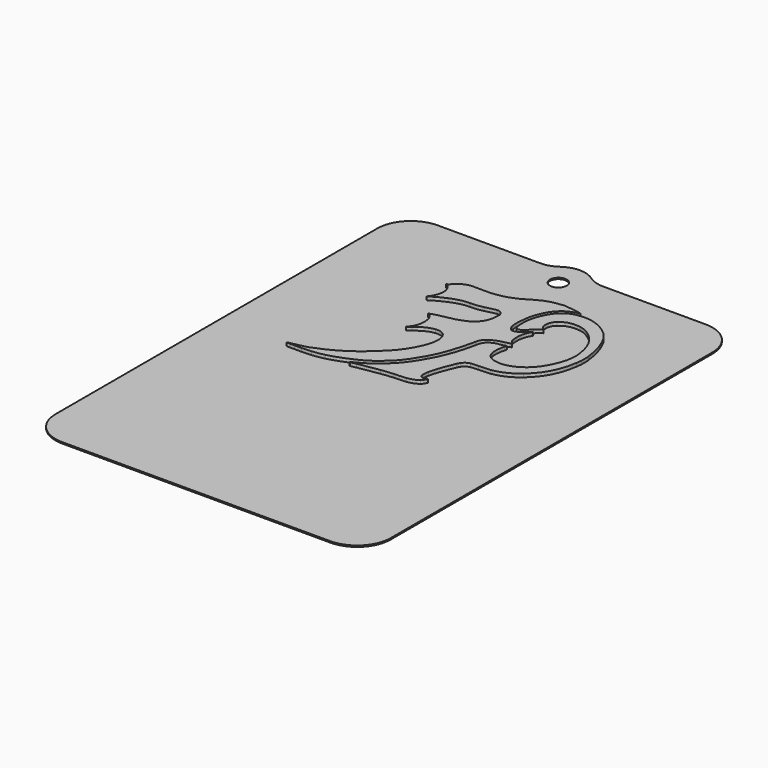
from build123d import *

# Parameters (mm, degrees)
F0_R     = 2.5
F1_DEPTH = 0.2
F3_DEPTH = 1


# Not quite as in the source:
# - ends of sketch curves that miss each other by under 0.0002 mm in the source are joined


with BuildPart() as f1:
    # F0 (on Top) → F1 (new body, symmetric)
    with BuildSketch(Plane.XY):
        with BuildLine():
            Line((-9.3273790531, 70), (-40, 70))
            ThreePointArc((-40, 70), (-47.0710678119, 67.0710678119), (-50, 60))
            Line((-50, 60), (-50, -60))
            ThreePointArc((-50, -60), (-47.0710678119, -67.0710678119), (-40, -70))
            Line((-40, -70), (40, -70))
            ThreePointArc((40, -70), (47.0710678119, -67.0710678119), (50, -60))
            Line((50, -60), (50, 60))
            ThreePointArc((50, 60), (47.0710678119, 67.0710678119), (40, 70))
            Line((40, 70), (9.3273790531, 70))
            ThreePointArc((9.3273790531, 70), (6.8778893103, 70.3842268941), (4.6636895265, 71.5))
            ThreePointArc((4.6636895265, 71.5), (0, 73), (-4.6636895265, 71.5))
            ThreePointArc((-4.6636895265, 71.5), (-6.8778893103, 70.3842268941), (-9.3273790531, 70))
        make_face()
        with Locations((0, 65)):
            Circle(F0_R, mode=Mode.SUBTRACT)
    extrude(amount=F1_DEPTH, both=True)

    # F2 (on face) → F3 (join)
    with BuildSketch(Plane.XY.offset(0.2)):
        with BuildLine():
            add(Edge.make_bspline(
                [(10.0940918419, 55.33162), (10.3944688419, 55.204597), (10.7172378419, 55.217338), (11.0315138419, 55.192628)],
                knots=[0, 0, 0, 0, 1, 1, 1, 1], degree=3))
            add(Edge.make_bspline(
                [(9.9539408419, 55.33162), (10.0006588419, 55.33162), (10.0473758419, 55.33162), (10.0940918419, 55.33162)],
                knots=[0, 0, 0, 0, 1, 1, 1, 1], degree=3))
            add(Edge.make_bspline(
                [(9.2528058419, 55.33162), (9.4867748419, 55.33162), (9.7203578419, 55.33162), (9.9539408419, 55.33162)],
                knots=[0, 0, 0, 0, 1, 1, 1, 1], degree=3))
            add(Edge.make_bspline(
                [(9.1829238419, 55.33162), (9.2060898419, 55.33162), (9.2296408419, 55.33162), (9.2528058419, 55.33162)],
                knots=[0, 0, 0, 0, 1, 1, 1, 1], degree=3))
            add(Edge.make_bspline(
                [(8.5254158419, 55.196103), (8.7489618419, 55.211932), (8.9786838419, 55.213091), (9.1829238419, 55.33162)],
                knots=[0, 0, 0, 0, 1, 1, 1, 1], degree=3))
            add(Edge.make_bspline(
                [(4.2919618419, 54.221617), (5.6490608419, 54.787622), (7.0652308419, 55.090315), (8.5254158419, 55.196103)],
                knots=[0, 0, 0, 0, 1, 1, 1, 1], degree=3))
            add(Edge.make_bspline(
                [(0.2326328419, 52.031726), (1.5545978419, 52.820503), (2.8676828419, 53.627427), (4.2919618419, 54.221617)],
                knots=[0, 0, 0, 0, 1, 1, 1, 1], degree=3))
            add(Edge.make_bspline(
                [(-9.8682011581, 49.538756), (-6.2826021581, 49.433354), (-2.8873441581, 50.170396), (0.2326328419, 52.031726)],
                knots=[0, 0, 0, 0, 1, 1, 1, 1], degree=3))
            add(Edge.make_bspline(
                [(-12.9140491581, 49.590491), (-11.8997961581, 49.615587), (-10.8839981581, 49.568484), (-9.8682011581, 49.538756)],
                knots=[0, 0, 0, 0, 1, 1, 1, 1], degree=3))
            add(Edge.make_bspline(
                [(-16.5571751581, 48.373542), (-15.5023831581, 49.256525), (-14.2402611581, 49.557674), (-12.9140491581, 49.590491)],
                knots=[0, 0, 0, 0, 1, 1, 1, 1], degree=3))
            add(Edge.make_bspline(
                [(-18.6961021581, 46.557384), (-17.8644691581, 47.043469), (-17.2695081581, 47.777808), (-16.5571751581, 48.373542)],
                knots=[0, 0, 0, 0, 1, 1, 1, 1], degree=3))
            add(Edge.make_bspline(
                [(-17.4463361581, 45.553555), (-17.7463261581, 46.02188), (-18.2092461581, 46.269363), (-18.6961021581, 46.557384)],
                knots=[0, 0, 0, 0, 1, 1, 1, 1], degree=3))
            add(Edge.make_bspline(
                [(-17.0818691581, 41.268751), (-16.6058231581, 42.730481), (-16.5726191581, 44.188734), (-17.4463361581, 45.553555)],
                knots=[0, 0, 0, 0, 1, 1, 1, 1], degree=3))
            add(Edge.make_bspline(
                [(-18.4300881581, 38.924039), (-17.8135051581, 39.617067), (-17.3610101581, 40.410864), (-17.0818691581, 41.268751)],
                knots=[0, 0, 0, 0, 1, 1, 1, 1], degree=3))
            add(Edge.make_bspline(
                [(-18.1783581581, 39.002415), (-18.2420631581, 38.957243), (-18.2972741581, 38.882728), (-18.4300881581, 38.924039)],
                knots=[0, 0, 0, 0, 1, 1, 1, 1], degree=3))
            add(Edge.make_bspline(
                [(-13.9483791581, 41.308132), (-15.4317291581, 40.67572), (-16.8583241581, 39.940608), (-18.1783581581, 39.002415)],
                knots=[0, 0, 0, 0, 1, 1, 1, 1], degree=3))
            add(Edge.make_bspline(
                [(-8.3779011581, 42.584153), (-10.3419311581, 42.619673), (-12.1650391581, 42.06834), (-13.9483791581, 41.308132)],
                knots=[0, 0, 0, 0, 1, 1, 1, 1], degree=3))
            add(Edge.make_bspline(
                [(-4.5328511581, 43.025065), (-5.8026941581, 42.745151), (-7.0806461581, 42.560987), (-8.3779011581, 42.584153)],
                knots=[0, 0, 0, 0, 1, 1, 1, 1], degree=3))
            add(Edge.make_bspline(
                [(-1.3754241581, 43.768671), (-2.4445011581, 43.591071), (-3.4765151581, 43.257876), (-4.5328511581, 43.025065)],
                knots=[0, 0, 0, 0, 1, 1, 1, 1], degree=3))
            add(Edge.make_bspline(
                [(0.7086788419, 42.071814), (0.6426578419, 43.163671), (-0.3221761581, 43.943955), (-1.3754241581, 43.768671)],
                knots=[0, 0, 0, 0, 1, 1, 1, 1], degree=3))
            add(Edge.make_bspline(
                [(0.5662128419, 40.378047), (0.6117708419, 40.942507), (0.7434268419, 41.498088), (0.7086788419, 42.071814)],
                knots=[0, 0, 0, 0, 1, 1, 1, 1], degree=3))
            add(Edge.make_bspline(
                [(-0.8874091581, 36.858468), (0.0237588419, 37.853803), (0.4588798419, 39.044499), (0.5662128419, 40.378047)],
                knots=[0, 0, 0, 0, 1, 1, 1, 1], degree=3))
            add(Edge.make_bspline(
                [(-3.3726571581, 35.005246), (-2.4024181581, 35.434962), (-1.6009001581, 36.078956), (-0.8874091581, 36.858468)],
                knots=[0, 0, 0, 0, 1, 1, 1, 1], degree=3))
            add(Edge.make_bspline(
                [(-5.8926531581, 34.088287), (-5.0316771581, 34.334997), (-4.1938661581, 34.641551), (-3.3726571581, 35.005246)],
                knots=[0, 0, 0, 0, 1, 1, 1, 1], degree=3))
            add(Edge.make_bspline(
                [(-10.8380541581, 33.021912), (-9.1917751581, 33.387537), (-7.5180831581, 33.622665), (-5.8926531581, 34.088287)],
                knots=[0, 0, 0, 0, 1, 1, 1, 1], degree=3))
            add(Edge.make_bspline(
                [(-12.7812341581, 32.350505), (-12.1495951581, 32.687946), (-11.4986501581, 32.875585), (-10.8380541581, 33.021912)],
                knots=[0, 0, 0, 0, 1, 1, 1, 1], degree=3))
            add(Edge.make_bspline(
                [(-11.0044581581, 30.218913), (-11.2191231581, 31.210001), (-11.8082931581, 31.929669), (-12.7812341581, 32.350505)],
                knots=[0, 0, 0, 0, 1, 1, 1, 1], degree=3))
            add(Edge.make_bspline(
                [(-12.5457211581, 24.119495), (-10.9013721581, 25.859207), (-10.5087211581, 27.931728), (-11.0044581581, 30.218913)],
                knots=[0, 0, 0, 0, 1, 1, 1, 1], degree=3))
            add(Edge.make_bspline(
                [(-12.5769951581, 23.968921), (-12.6275721581, 24.070462), (-12.5727451581, 24.091311), (-12.5457211581, 24.119495)],
                knots=[0, 0, 0, 0, 1, 1, 1, 1], degree=3))
            add(Edge.make_bspline(
                [(-11.5044411581, 24.802099), (-11.8654341581, 24.534153), (-12.2152301581, 24.250379), (-12.5769951581, 23.968921)],
                knots=[0, 0, 0, 0, 1, 1, 1, 1], degree=3))
            add(Edge.make_bspline(
                [(-6.4984251581, 27.232909), (-8.4358151581, 26.997009), (-9.9859581581, 25.92909), (-11.5044411581, 24.802099)],
                knots=[0, 0, 0, 0, 1, 1, 1, 1], degree=3))
            add(Edge.make_bspline(
                [(-2.7190101581, 24.706735), (-3.2228551581, 26.661885), (-4.5575611581, 27.469195), (-6.4984251581, 27.232909)],
                knots=[0, 0, 0, 0, 1, 1, 1, 1], degree=3))
            add(Edge.make_bspline(
                [(-2.7722901581, 21.715325), (-2.5653471581, 22.709502), (-2.4703691581, 23.741901), (-2.7190101581, 24.706735)],
                knots=[0, 0, 0, 0, 1, 1, 1, 1], degree=3))
            add(Edge.make_bspline(
                [(-5.7428511581, 15.177312), (-4.4170251581, 17.193077), (-3.2742041581, 19.308453), (-2.7722901581, 21.715325)],
                knots=[0, 0, 0, 0, 1, 1, 1, 1], degree=3))
            add(Edge.make_bspline(
                [(-11.4341741581, 9.089477), (-9.3361711581, 10.922622), (-7.2918361581, 12.822175), (-5.7428511581, 15.177312)],
                knots=[0, 0, 0, 0, 1, 1, 1, 1], degree=3))
            add(Edge.make_bspline(
                [(-14.5618731581, 6.584538), (-13.4534141581, 7.317333), (-12.4407051581, 8.209968), (-11.4341741581, 9.089477)],
                knots=[0, 0, 0, 0, 1, 1, 1, 1], degree=3))
            add(Edge.make_bspline(
                [(-18.2134931581, 4.309321), (-16.9239591581, 4.957948), (-15.7556561581, 5.79576), (-14.5618731581, 6.584538)],
                knots=[0, 0, 0, 0, 1, 1, 1, 1], degree=3))
            add(Edge.make_bspline(
                [(-21.1991111581, 2.868823), (-20.1566731581, 3.238313), (-19.2018781581, 3.812426), (-18.2134931581, 4.309321)],
                knots=[0, 0, 0, 0, 1, 1, 1, 1], degree=3))
            add(Edge.make_bspline(
                [(-24.0897521581, 1.666931), (-23.0890121581, 1.970396), (-22.1859521581, 2.519027), (-21.1991111581, 2.868823)],
                knots=[0, 0, 0, 0, 1, 1, 1, 1], degree=3))
            add(Edge.make_bspline(
                [(-25.6128691581, 1.290496), (-25.1070931581, 1.424467), (-24.5897361581, 1.515585), (-24.0897521581, 1.666931)],
                knots=[0, 0, 0, 0, 1, 1, 1, 1], degree=3))
            add(Edge.make_bspline(
                [(-29.4328231581, 0.475463), (-28.1529421581, 0.71561), (-26.8734461581, 0.956916), (-25.6128691581, 1.290496)],
                knots=[0, 0, 0, 0, 1, 1, 1, 1], degree=3))
            add(Edge.make_bspline(
                [(-29.4328231581, 0.475463), (-29.0664261581, 0.330298), (-28.6830401581, 0.464657), (-28.3116241581, 0.404814)],
                knots=[0, 0, 0, 0, 1, 1, 1, 1], degree=3))
            Line((-28.3116241581, 0.404814), (-27.0529771581, 0.404042))
            add(Edge.make_bspline(
                [(-26.6325271581, 0.404042), (-26.7726771581, 0.404042), (-26.9128271581, 0.404042), (-27.0529771581, 0.404042)],
                knots=[0, 0, 0, 0, 1, 1, 1, 1], degree=3))
            add(Edge.make_bspline(
                [(-25.9313911581, 0.404042), (-26.1653601581, 0.404042), (-26.3989431581, 0.404042), (-26.6325271581, 0.404042)],
                knots=[0, 0, 0, 0, 1, 1, 1, 1], degree=3))
            add(Edge.make_bspline(
                [(-24.9503421581, 0.404042), (-25.2773581581, 0.404042), (-25.6043751581, 0.404042), (-25.9313911581, 0.404042)],
                knots=[0, 0, 0, 0, 1, 1, 1, 1], degree=3))
            add(Edge.make_bspline(
                [(-22.0855691581, 0.557318), (-23.0384341581, 0.460024), (-23.9928441581, 0.402883), (-24.9503421581, 0.404042)],
                knots=[0, 0, 0, 0, 1, 1, 1, 1], degree=3))
            add(Edge.make_bspline(
                [(-18.5343311581, 1.110968), (-19.6949121581, 0.813681), (-20.8917851581, 0.679708), (-22.0855691581, 0.557318)],
                knots=[0, 0, 0, 0, 1, 1, 1, 1], degree=3))
            add(Edge.make_bspline(
                [(-10.4612321581, 4.162221), (-13.0646231581, 2.913227), (-15.7359661581, 1.827161), (-18.5343311581, 1.110968)],
                knots=[0, 0, 0, 0, 1, 1, 1, 1], degree=3))
            add(Edge.make_bspline(
                [(-4.8602541581, 8.231975), (-6.5744851581, 6.655192), (-8.3562801581, 5.171842), (-10.4612321581, 4.162221)],
                knots=[0, 0, 0, 0, 1, 1, 1, 1], degree=3))
            add(Edge.make_bspline(
                [(0.3469148419, 15.298543), (-1.1252391581, 12.748818), (-2.6699771581, 10.246968), (-4.8602541581, 8.231975)],
                knots=[0, 0, 0, 0, 1, 1, 1, 1], degree=3))
            add(Edge.make_bspline(
                [(2.8645938419, 21.104535), (2.1846938419, 19.099193), (1.4044088419, 17.129758), (0.3469148419, 15.298543)],
                knots=[0, 0, 0, 0, 1, 1, 1, 1], degree=3))
            add(Edge.make_bspline(
                [(4.7807488419, 28.180755), (4.2896448419, 25.779674), (3.6502828419, 23.421835), (2.8645938419, 21.104535)],
                knots=[0, 0, 0, 0, 1, 1, 1, 1], degree=3))
            add(Edge.make_bspline(
                [(6.2444078419, 30.588786), (5.4015788419, 30.001159), (4.9772678419, 29.142499), (4.7807488419, 28.180755)],
                knots=[0, 0, 0, 0, 1, 1, 1, 1], degree=3))
            add(Edge.make_bspline(
                [(9.5157318419, 32.030438), (8.3466578419, 31.73508), (7.2443758419, 31.285674), (6.2444078419, 30.588786)],
                knots=[0, 0, 0, 0, 1, 1, 1, 1], degree=3))
            add(Edge.make_bspline(
                [(11.5388328419, 32.54934), (10.8913638419, 32.270585), (10.1906138419, 32.201089), (9.5157318419, 32.030438)],
                knots=[0, 0, 0, 0, 1, 1, 1, 1], degree=3))
            add(Edge.make_bspline(
                [(11.6554318419, 33.103376), (12.0129498419, 32.764777), (12.0005948419, 32.74779), (11.5388328419, 32.54934)],
                knots=[0, 0, 0, 0, 1, 1, 1, 1], degree=3))
            add(Edge.make_bspline(
                [(11.0071888419, 34.327661), (11.0901988419, 33.855476), (11.2983008419, 33.442362), (11.6554318419, 33.103376)],
                knots=[0, 0, 0, 0, 1, 1, 1, 1], degree=3))
            add(Edge.make_bspline(
                [(11.9492438419, 40.017054), (10.8600898419, 38.25186), (10.6531468419, 36.335705), (11.0071888419, 34.327661)],
                knots=[0, 0, 0, 0, 1, 1, 1, 1], degree=3))
            add(Edge.make_bspline(
                [(12.1040658419, 40.391945), (12.1110138419, 40.195427), (12.0079298419, 40.112032), (11.9492438419, 40.017054)],
                knots=[0, 0, 0, 0, 1, 1, 1, 1], degree=3))
            add(Edge.make_bspline(
                [(11.4863248419, 39.735982), (11.6909508419, 39.926323), (11.8716408419, 40.143305), (12.1040658419, 40.391945)],
                knots=[0, 0, 0, 0, 1, 1, 1, 1], degree=3))
            add(Edge.make_bspline(
                [(8.9420048419, 38.025998), (9.9168768419, 38.407454), (10.7284338419, 39.02944), (11.4863248419, 39.735982)],
                knots=[0, 0, 0, 0, 1, 1, 1, 1], degree=3))
            add(Edge.make_bspline(
                [(6.7922668419, 38.884658), (7.2076978419, 38.142597), (7.8208058419, 37.587016), (8.9420048419, 38.025998)],
                knots=[0, 0, 0, 0, 1, 1, 1, 1], degree=3))
            add(Edge.make_bspline(
                [(6.5173728419, 39.716678), (6.5733558419, 39.425953), (6.6467128419, 39.145267), (6.7922668419, 38.884658)],
                knots=[0, 0, 0, 0, 1, 1, 1, 1], degree=3))
            add(Edge.make_bspline(
                [(6.6289518419, 44.590652), (6.4297298419, 42.977962), (6.2030978419, 41.349443), (6.5173728419, 39.716678)],
                knots=[0, 0, 0, 0, 1, 1, 1, 1], degree=3))
            add(Edge.make_bspline(
                [(8.1408718419, 49.376985), (7.3683108419, 47.868925), (6.8358948419, 46.267818), (6.6289518419, 44.590652)],
                knots=[0, 0, 0, 0, 1, 1, 1, 1], degree=3))
            add(Edge.make_bspline(
                [(13.1163888419, 53.981856), (10.7983158419, 53.173002), (9.2427678419, 51.528267), (8.1408718419, 49.376985)],
                knots=[0, 0, 0, 0, 1, 1, 1, 1], degree=3))
            add(Edge.make_bspline(
                [(15.1031968419, 54.423927), (14.4020608419, 54.402692), (13.7592248419, 54.205787), (13.1163888419, 53.981856)],
                knots=[0, 0, 0, 0, 1, 1, 1, 1], degree=3))
            add(Edge.make_bspline(
                [(14.7896938419, 54.609635), (14.8916218419, 54.583381), (15.0255928419, 54.58647), (15.1031968419, 54.423927)],
                knots=[0, 0, 0, 0, 1, 1, 1, 1], degree=3))
            add(Edge.make_bspline(
                [(11.0315138419, 55.192628), (12.2990408419, 55.092631), (13.5553698419, 54.924683), (14.7896938419, 54.609635)],
                knots=[0, 0, 0, 0, 1, 1, 1, 1], degree=3))
        make_face()
        with BuildLine():
            add(Edge.make_bspline(
                [(30.0000158419, 35.937262), (29.8228008419, 35.509091), (29.8656578419, 35.046557), (29.8042688419, 34.601398)],
                knots=[0, 0, 0, 0, 1, 1, 1, 1], degree=3))
            add(Edge.make_bspline(
                [(30.0000158419, 36.363504), (30.0000158419, 36.221423), (30.0000158419, 36.079343), (30.0000158419, 35.937262)],
                knots=[0, 0, 0, 0, 1, 1, 1, 1], degree=3))
            add(Edge.make_bspline(
                [(30.0000158419, 36.505584), (30.0000158419, 36.458095), (30.0000158419, 36.410993), (30.0000158419, 36.363504)],
                knots=[0, 0, 0, 0, 1, 1, 1, 1], degree=3))
            add(Edge.make_bspline(
                [(30.0000158419, 36.860785), (30.0000158419, 36.742256), (30.0000158419, 36.624113), (30.0000158419, 36.505584)],
                knots=[0, 0, 0, 0, 1, 1, 1, 1], degree=3))
            add(Edge.make_bspline(
                [(30.0000158419, 37.784307), (30.0000158419, 37.476595), (30.0000158419, 37.168497), (30.0000158419, 36.860785)],
                knots=[0, 0, 0, 0, 1, 1, 1, 1], degree=3))
            add(Edge.make_bspline(
                [(30.0000158419, 38.565749), (30.0000158419, 38.30514), (30.0000158419, 38.044917), (30.0000158419, 37.784307)],
                knots=[0, 0, 0, 0, 1, 1, 1, 1], degree=3))
            add(Edge.make_bspline(
                [(29.8629538419, 39.122874), (29.8868918419, 38.934849), (29.8737648419, 38.730609), (30.0000158419, 38.565749)],
                knots=[0, 0, 0, 0, 1, 1, 1, 1], degree=3))
            add(Edge.make_bspline(
                [(28.6668538419, 44.452819), (29.3015818419, 42.730481), (29.6340048419, 40.939032), (29.8629538419, 39.122874)],
                knots=[0, 0, 0, 0, 1, 1, 1, 1], degree=3))
            add(Edge.make_bspline(
                [(25.3001668419, 50.121748), (27.0016558419, 48.587821), (27.8919758419, 46.554296), (28.6668538419, 44.452819)],
                knots=[0, 0, 0, 0, 1, 1, 1, 1], degree=3))
            add(Edge.make_bspline(
                [(14.4815958419, 53.337089), (18.6386048419, 54.179919), (22.1952478419, 52.920886), (25.3001668419, 50.121748)],
                knots=[0, 0, 0, 0, 1, 1, 1, 1], degree=3))
            add(Edge.make_bspline(
                [(10.5635748419, 51.03446), (11.6326528419, 52.218592), (12.9229588419, 53.020883), (14.4815958419, 53.337089)],
                knots=[0, 0, 0, 0, 1, 1, 1, 1], degree=3))
            add(Edge.make_bspline(
                [(8.3848798419, 47.353112), (8.9134348419, 48.693609), (9.5906328419, 49.956503), (10.5635748419, 51.03446)],
                knots=[0, 0, 0, 0, 1, 1, 1, 1], degree=3))
            add(Edge.make_bspline(
                [(7.5100048419, 40.679195), (7.2771938419, 42.972557), (7.5389618419, 45.208778), (8.3848798419, 47.353112)],
                knots=[0, 0, 0, 0, 1, 1, 1, 1], degree=3))
            add(Edge.make_bspline(
                [(7.8582558419, 39.613978), (7.6513128419, 39.936362), (7.5478408419, 40.30662), (7.5100048419, 40.679195)],
                knots=[0, 0, 0, 0, 1, 1, 1, 1], degree=3))
            add(Edge.make_bspline(
                [(8.2018738419, 39.285803), (8.0292938419, 39.293137), (7.9451268419, 39.478847), (7.8582558419, 39.613978)],
                knots=[0, 0, 0, 0, 1, 1, 1, 1], degree=3))
            add(Edge.make_bspline(
                [(9.3107188419, 39.482323), (8.9516578419, 39.240245), (8.5806268419, 39.269974), (8.2018738419, 39.285803)],
                knots=[0, 0, 0, 0, 1, 1, 1, 1], degree=3))
            add(Edge.make_bspline(
                [(11.4334308419, 41.377628), (10.7809418419, 40.68267), (10.1060608419, 40.018212), (9.3107188419, 39.482323)],
                knots=[0, 0, 0, 0, 1, 1, 1, 1], degree=3))
            add(Edge.make_bspline(
                [(13.2322148419, 42.848623), (12.5210408419, 42.508479), (11.9712518419, 41.950197), (11.4334308419, 41.377628)],
                knots=[0, 0, 0, 0, 1, 1, 1, 1], degree=3))
            add(Edge.make_bspline(
                [(12.5662128419, 43.547056), (12.7828088419, 43.316176), (13.0032648419, 43.08877), (13.2322148419, 42.848623)],
                knots=[0, 0, 0, 0, 1, 1, 1, 1], degree=3))
            add(Edge.make_bspline(
                [(12.2164178419, 44.151284), (12.2492348419, 43.920017), (12.4036698419, 43.720796), (12.5662128419, 43.547056)],
                knots=[0, 0, 0, 0, 1, 1, 1, 1], degree=3))
            add(Edge.make_bspline(
                [(13.3275788419, 47.779353), (12.2666088419, 46.82031), (12.0183538419, 45.535795), (12.2164178419, 44.151284)],
                knots=[0, 0, 0, 0, 1, 1, 1, 1], degree=3))
            add(Edge.make_bspline(
                [(19.0571248419, 49.253823), (16.9564198419, 49.568098), (14.9696108419, 49.263475), (13.3275788419, 47.779353)],
                knots=[0, 0, 0, 0, 1, 1, 1, 1], degree=3))
            add(Edge.make_bspline(
                [(22.8473498419, 47.46778), (21.7273088419, 48.336864), (20.4829468419, 49.040702), (19.0571248419, 49.253823)],
                knots=[0, 0, 0, 0, 1, 1, 1, 1], degree=3))
            add(Edge.make_bspline(
                [(27.4529938419, 38.2646), (27.0549368419, 41.886106), (25.8244748419, 45.157429), (22.8473498419, 47.46778)],
                knots=[0, 0, 0, 0, 1, 1, 1, 1], degree=3))
            add(Edge.make_bspline(
                [(25.8661718419, 30.464079), (27.0703808419, 32.921916), (27.7545278419, 35.523762), (27.4529938419, 38.2646)],
                knots=[0, 0, 0, 0, 1, 1, 1, 1], degree=3))
            add(Edge.make_bspline(
                [(20.5489688419, 24.472379), (22.9894298419, 25.852258), (24.6434308419, 27.968407), (25.8661718419, 30.464079)],
                knots=[0, 0, 0, 0, 1, 1, 1, 1], degree=3))
            add(Edge.make_bspline(
                [(14.1568948419, 23.435733), (16.4309528419, 22.88247), (18.5498038419, 23.341528), (20.5489688419, 24.472379)],
                knots=[0, 0, 0, 0, 1, 1, 1, 1], degree=3))
            add(Edge.make_bspline(
                [(11.2600778419, 26.561888), (11.4990658419, 24.843024), (12.5121608419, 23.836106), (14.1568948419, 23.435733)],
                knots=[0, 0, 0, 0, 1, 1, 1, 1], degree=3))
            add(Edge.make_bspline(
                [(11.6006068419, 30.382228), (11.2677988419, 29.127829), (11.0797748419, 27.856827), (11.2600778419, 26.561888)],
                knots=[0, 0, 0, 0, 1, 1, 1, 1], degree=3))
            add(Edge.make_bspline(
                [(11.7700988419, 31.117726), (11.7924928419, 30.834724), (11.6623808419, 30.615039), (11.6006068419, 30.382228)],
                knots=[0, 0, 0, 0, 1, 1, 1, 1], degree=3))
            add(Edge.make_bspline(
                [(10.0122408419, 30.63666), (10.6110628419, 30.717738), (11.2006198419, 30.835882), (11.7700988419, 31.117726)],
                knots=[0, 0, 0, 0, 1, 1, 1, 1], degree=3))
            add(Edge.make_bspline(
                [(9.2867808419, 30.534733), (9.5234538419, 30.590716), (9.7701638419, 30.603843), (10.0122408419, 30.63666)],
                knots=[0, 0, 0, 0, 1, 1, 1, 1], degree=3))
            add(Edge.make_bspline(
                [(6.2556058419, 28.318588), (6.8814538419, 29.600786), (7.9733098419, 30.224704), (9.2867808419, 30.534733)],
                knots=[0, 0, 0, 0, 1, 1, 1, 1], degree=3))
            add(Edge.make_bspline(
                [(5.8004078419, 26.511697), (5.9254998419, 27.122102), (5.9764638419, 27.747178), (6.2556058419, 28.318588)],
                knots=[0, 0, 0, 0, 1, 1, 1, 1], degree=3))
            add(Edge.make_bspline(
                [(0.6472908419, 13.165021), (3.2113008419, 17.277631), (4.8274658419, 21.76822), (5.8004078419, 26.511697)],
                knots=[0, 0, 0, 0, 1, 1, 1, 1], degree=3))
            add(Edge.make_bspline(
                [(-2.7139901581, 8.520769), (-1.4051531581, 9.946205), (-0.3661901581, 11.538433), (0.6472908419, 13.165021)],
                knots=[0, 0, 0, 0, 1, 1, 1, 1], degree=3))
            add(Edge.make_bspline(
                [(-11.7669811581, 1.895113), (-8.2879431581, 3.456067), (-5.3077301581, 5.694991), (-2.7139901581, 8.520769)],
                knots=[0, 0, 0, 0, 1, 1, 1, 1], degree=3))
            add(Edge.make_bspline(
                [(-11.7669811581, 1.895113), (-11.7187201581, 1.872333), (-11.6708461581, 1.849169), (-11.6225851581, 1.826389)],
                knots=[0, 0, 0, 0, 1, 1, 1, 1], degree=3))
            add(Edge.make_bspline(
                [(-9.9164621581, 2.184679), (-10.4909611581, 2.097423), (-11.0422941581, 1.890866), (-11.6225851581, 1.826389)],
                knots=[0, 0, 0, 0, 1, 1, 1, 1], degree=3))
            add(Edge.make_bspline(
                [(-3.6097141581, 3.226344), (-5.7254771581, 2.964577), (-7.8095801581, 2.505518), (-9.9164621581, 2.184679)],
                knots=[0, 0, 0, 0, 1, 1, 1, 1], degree=3))
            add(Edge.make_bspline(
                [(0.1121738419, 3.61166), (-1.1360491581, 3.572279), (-2.3715311581, 3.379621), (-3.6097141581, 3.226344)],
                knots=[0, 0, 0, 0, 1, 1, 1, 1], degree=3))
            add(Edge.make_bspline(
                [(3.6051108419, 3.824781), (2.4449168419, 3.674979), (1.2793168419, 3.648338), (0.1121738419, 3.61166)],
                knots=[0, 0, 0, 0, 1, 1, 1, 1], degree=3))
            add(Edge.make_bspline(
                [(6.8046218419, 5.023198), (5.8525288419, 4.301213), (4.7649188419, 3.974583), (3.6051108419, 3.824781)],
                knots=[0, 0, 0, 0, 1, 1, 1, 1], degree=3))
            add(Edge.make_bspline(
                [(7.8547808419, 6.676426), (7.6594208419, 5.989962), (7.3513228419, 5.437084), (6.8046218419, 5.023198)],
                knots=[0, 0, 0, 0, 1, 1, 1, 1], degree=3))
            add(Edge.make_bspline(
                [(7.2200528419, 6.403848), (7.4227488419, 6.479136), (7.6181088419, 6.574114), (7.8547808419, 6.676426)],
                knots=[0, 0, 0, 0, 1, 1, 1, 1], degree=3))
            add(Edge.make_bspline(
                [(5.5409568419, 7.545125), (5.5915338419, 6.535119), (6.2899668419, 6.057527), (7.2200528419, 6.403848)],
                knots=[0, 0, 0, 0, 1, 1, 1, 1], degree=3))
            add(Edge.make_bspline(
                [(5.7119938419, 9.410316), (5.5753178419, 8.796822), (5.5092968419, 8.175606), (5.5409568419, 7.545125)],
                knots=[0, 0, 0, 0, 1, 1, 1, 1], degree=3))
            add(Edge.make_bspline(
                [(8.2945358419, 16.820116), (7.2849158419, 14.403591), (6.2837888419, 11.983592), (5.7119938419, 9.410316)],
                knots=[0, 0, 0, 0, 1, 1, 1, 1], degree=3))
            add(Edge.make_bspline(
                [(8.7103518419, 17.554841), (8.5539868419, 17.321644), (8.4026398419, 17.078409), (8.2945358419, 16.820116)],
                knots=[0, 0, 0, 0, 1, 1, 1, 1], degree=3))
            add(Edge.make_bspline(
                [(10.6797868419, 18.905378), (9.8292358419, 18.727777), (9.1875568419, 18.268718), (8.7103518419, 17.554841)],
                knots=[0, 0, 0, 0, 1, 1, 1, 1], degree=3))
            add(Edge.make_bspline(
                [(12.9414908419, 19.086066), (12.1890058419, 19.05711), (11.4291848419, 19.062129), (10.6797868419, 18.905378)],
                knots=[0, 0, 0, 0, 1, 1, 1, 1], degree=3))
            add(Edge.make_bspline(
                [(16.4313398419, 19.267913), (15.2769368419, 19.082591), (14.1059318419, 19.131238), (12.9414908419, 19.086066)],
                knots=[0, 0, 0, 0, 1, 1, 1, 1], degree=3))
            add(Edge.make_bspline(
                [(23.5287948419, 22.594447), (21.4778948419, 20.818829), (19.1034548419, 19.696858), (16.4313398419, 19.267913)],
                knots=[0, 0, 0, 0, 1, 1, 1, 1], degree=3))
            add(Edge.make_bspline(
                [(29.8042688419, 34.601398), (29.1479198419, 29.825876), (27.1765538419, 25.752648), (23.5287948419, 22.594447)],
                knots=[0, 0, 0, 0, 1, 1, 1, 1], degree=3))
        make_face()
    extrude(amount=F3_DEPTH)


solid = f1.part
